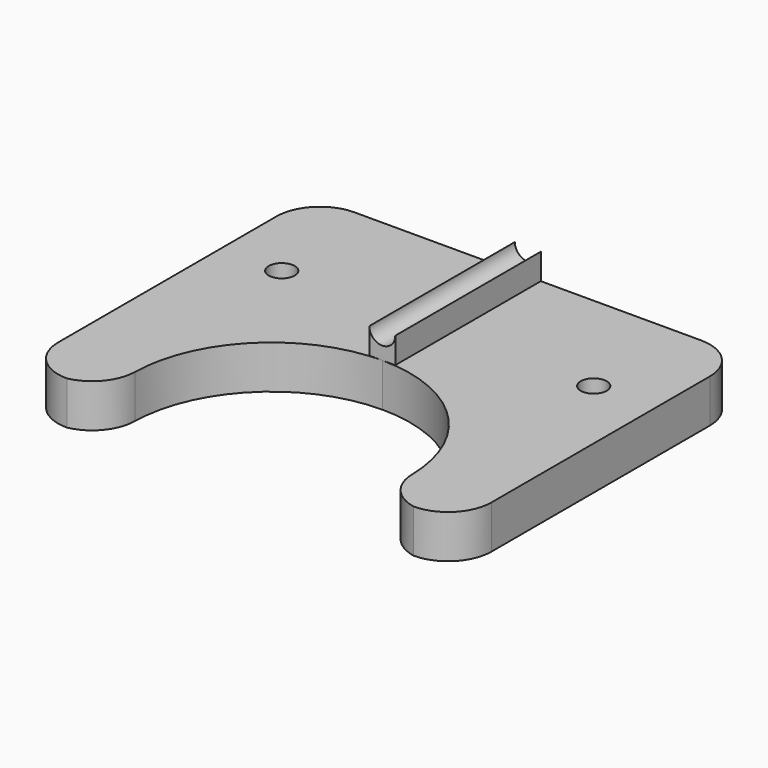
from build123d import *

# Parameters (mm, degrees)
F0_R        = 1.5
F1_DEPTH    = 5
F2_R        = 5
F3_W        = 3
F3_H        = 21
F4_DEPTH    = 3
F5_R        = 1.5
F6_DEPTH    = 21
F7_T1_DEPTH = 29.0228793414


# Not quite as in the source:
# - a fillet or chamfer that OpenCascade refuses, or shapes differently, is made with other operations: its cross-section is extruded or revolved along the edge and cut away or added


with BuildPart() as f1:
    # F0 (on Top) → F1 (new body)
    with BuildSketch(Plane.XY):
        Polygon((0, -10.5), (25, -10.5), (25, 10.5), (-25, 10.5), (-25, -10.5), align=None)
        with Locations((-18, -2.5)):
            Circle(F0_R, mode=Mode.SUBTRACT)
        with Locations((18, -2.5)):
            Circle(F0_R, mode=Mode.SUBTRACT)
        with BuildLine():
            Line((25, -31), (25, -10.5))
            Line((25, -10.5), (0, -10.5))
            ThreePointArc((0, -10.5), (11.313708499, -15.186291501), (16, -26.5))
            Line((16, -26.5), (16, -31))
            Line((16, -31), (25, -31))
        make_face()
        with BuildLine():
            ThreePointArc((-16, -26.5), (-11.313708499, -15.186291501), (0, -10.5))
            Line((0, -10.5), (-25, -10.5))
            Line((-25, -10.5), (-25, -31))
            Line((-25, -31), (-16, -31))
            Line((-16, -31), (-16, -26.5))
        make_face()
    extrude(amount=F1_DEPTH)

    # F2
    f2_edges = [f1.edges().sort_by_distance(p)[0] for p in [
        (25, -31, 2.5),
        (-25, -31, 2.5),
        (-25, 10.5, 2.5),
        (25, 10.5, 2.5),
    ]]
    fillet(f2_edges, radius=F2_R)

    # F3 (on face) → F4 (join)
    with BuildSketch(Plane.XY.offset(5)):
        Rectangle(F3_W, F3_H)
    extrude(amount=F4_DEPTH)

    # F5 (on face) → F6 (cut, through all)
    with BuildSketch(Plane(origin=(0, 10.5, 0), x_dir=(-1, 0, 0), z_dir=(0, 1, 0))):
        with Locations((0, 8)):
            Circle(F5_R)
    extrude(amount=-F6_DEPTH, mode=Mode.SUBTRACT)

    # F7: fillet of radius 5 on 2 edges, made by hand

    # F7_s2 → F7_t1 (cut)
    with BuildSketch(Plane.XY.offset(-12.0114396707)):
        with BuildLine():
            ThreePointArc((20, -31), (17.1547293043, -29.3007363495), (15.9971008021, -26.1954250064))
            Line((15.9971008021, -26.1954250064), (15.4971914021, -26.204942975))
            ThreePointArc((15.4971914021, -26.204942975), (15.5, -26.5), (15.5, -31))
            Line((15.5, -31), (16, -31.5))
            ThreePointArc((16, -31.5), (18, -31.5), (19.9003805197, -31.4899754679))
            Line((19.9003805197, -31.4899754679), (20, -31))
        make_face()
        with BuildLine():
            ThreePointArc((-20, -31), (-17.1547293043, -29.3007363495), (-15.9971008021, -26.1954250064))
            Line((-15.9971008021, -26.1954250064), (-15.4971914021, -26.204942975))
            ThreePointArc((-15.4971914021, -26.204942975), (-15.5, -26.5), (-15.5, -31))
            Line((-15.5, -31), (-16, -31.5))
            ThreePointArc((-16, -31.5), (-18, -31.5), (-19.9003805197, -31.4899754679))
            Line((-19.9003805197, -31.4899754679), (-20, -31))
        make_face()
    extrude(amount=F7_T1_DEPTH, mode=Mode.SUBTRACT)


solid = f1.part
